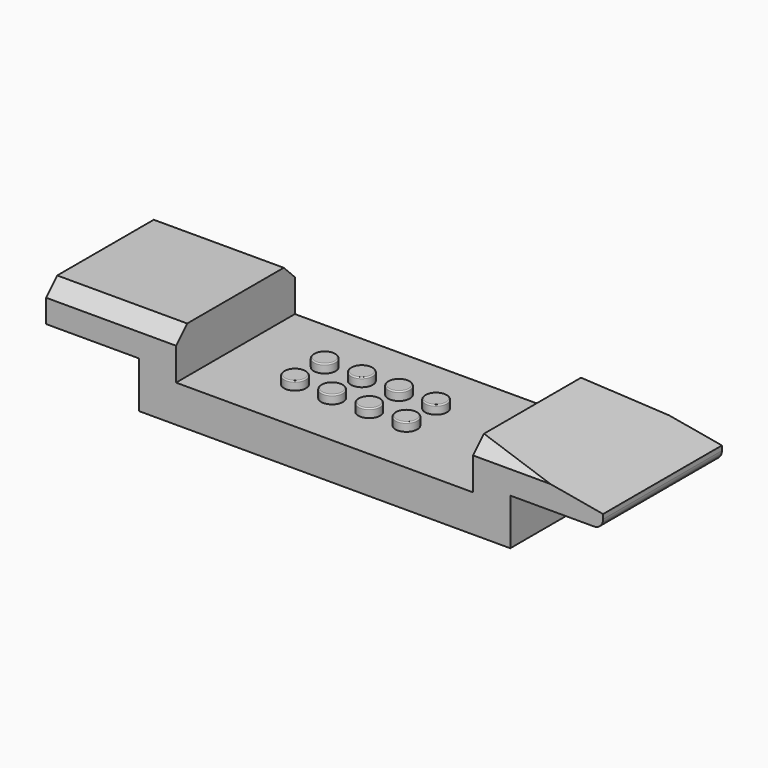
from build123d import *

# Parameters (mm, degrees)
F1_DEPTH    = 32
F2_W        = 13.0169491525
F2_H        = 29.0338983051
F2_R        = 3.2542372881
F2_R_2      = 2.4025423729
F3_DEPTH    = 3.5
F5_R        = 2.3495
F6_DEPTH    = 1.85
F7_SIZE     = 3
F8_R        = 2
F9_T1_DEPTH = 173.3704583371
F10_R       = 0.25


# Not quite as in the source:
# - a fillet or chamfer that OpenCascade refuses, or shapes differently, is made with other operations: its cross-section is extruded or revolved along the edge and cut away or added


with BuildPart() as f1:
    # F0 (on Front) → F1 (new body)
    with BuildSketch(Plane.XZ):
        Polygon((-40, 0), (0, 0), (0, 8), (-32, 8), (-32, 18), (-60, 18), (-60, 10), (-40, 10), align=None)
    extrude(amount=-F1_DEPTH)

    # F2 (on face) → F3 (cut)
    with BuildSketch(Plane(origin=(0, 0, 10), x_dir=(1, 0, 0), z_dir=(0, 0, -1))):
        with Locations((-50, -15.9830508475)):
            Rectangle(F2_W, F2_H)
        with Locations((-50, -23.9915254237)):
            Circle(F2_R, mode=Mode.SUBTRACT)
        with Locations((-50, -15.9830508475)):
            Circle(F2_R, mode=Mode.SUBTRACT)
        with Locations((-50, -7.9745762712)):
            Circle(F2_R, mode=Mode.SUBTRACT)
        with Locations((-50, -15.9830508475)):
            Circle(F2_R_2)
        with Locations((-50, -7.9745762712)):
            Circle(F2_R_2)
        with Locations((-50, -23.9915254237)):
            Circle(F2_R_2)
    extrude(amount=-F3_DEPTH, mode=Mode.SUBTRACT)

    # F4: F1 across face


with BuildPart() as f1_1:
    add(f1.part)
    add(f1.part.mirror(Plane(origin=(0, 16, 4), x_dir=(0, 1, 0), z_dir=(1, 0, 0))))

    # F5 (on face) → F6 (join)
    with BuildSketch(Plane.XY.offset(8)):
        with Locations((-16.002, 12.0333669113)):
            Circle(F5_R)
        with Locations((-16.002, 20.0343669113)):
            Circle(F5_R)
        with Locations((-8.001, 20.0343669113)):
            Circle(F5_R)
        with Locations((-8.001, 12.0333669113)):
            Circle(F5_R)
        with Locations((0, 12.0333669113)):
            Circle(F5_R)
        with Locations((0, 20.0343669113)):
            Circle(F5_R)
        with Locations((8.001, 20.0343669113)):
            Circle(F5_R)
        with Locations((8.001, 12.0333669113)):
            Circle(F5_R)
    extrude(amount=F6_DEPTH)

    # F7
    f7_edges = [f1_1.edges().sort_by_distance(p)[0] for p in [
        (-46, 0, 18),
        (-46, 32, 18),
        (46, 0, 18),
        (46, 32, 18),
    ]]
    chamfer(f7_edges, length=F7_SIZE)

    # F8
    f8_edges = [f1_1.edges().sort_by_distance(p)[0] for p in [
        (60, 16, 10),
    ]]
    fillet(f8_edges, radius=F8_R)

    # F9: chamfer of 5 x 28.3564090981 on 1 edges, made by hand

    # F9_s2 → F9_t1 (cut)
    with BuildSketch(Plane.XZ.offset(-102.6852291686)):
        Polygon((60, 13), (31.6435909019, 18), (60, 18), align=None)
    extrude(amount=F9_T1_DEPTH, mode=Mode.SUBTRACT)

    # F10
    f10_edges = [f1_1.edges().sort_by_distance(p)[0] for p in [
        (-18.3515, 12.033367, 9.85),
        (-18.3515, 20.034367, 9.85),
        (-10.3505, 20.034367, 9.85),
        (-10.3505, 12.033367, 9.85),
        (-2.3495, 12.033367, 9.85),
        (5.6515, 12.033367, 9.85),
        (5.6515, 20.034367, 9.85),
        (-2.3495, 20.034367, 9.85),
    ]]
    fillet(f10_edges, radius=F10_R)


solid = f1_1.part
